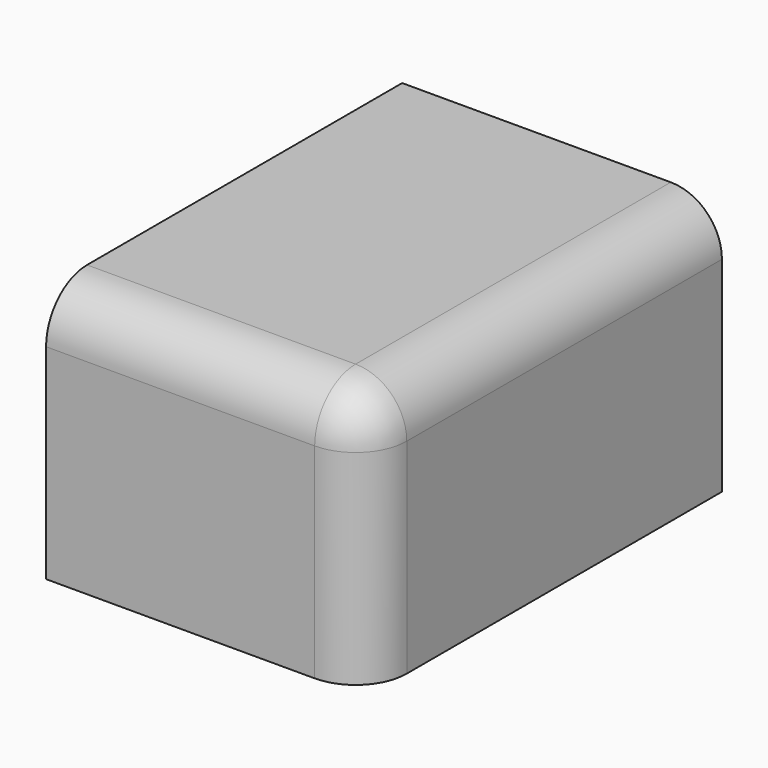
from build123d import *

# Parameters (mm, degrees)
F0_W        = 31.75
F0_H        = 25.4
F1_DEPTH    = 44.196
F2_R        = 5.08
F3_T1_DEPTH = 33.02
F3_S5_W     = 5.08
F3_S5_H     = 5.08
F3_T6_DEPTH = 5.08


# Not quite as in the source:
# - a fillet or chamfer that OpenCascade refuses, or shapes differently, is made with other operations: its cross-section is extruded or revolved along the edge and cut away or added


with BuildPart() as f1:
    # F0 (on Front) → F1 (new body)
    with BuildSketch(Plane.XZ):
        with Locations((3.175, 0)):
            Rectangle(F0_W, F0_H)
    extrude(amount=F1_DEPTH)

    # F2
    f2_edges = [f1.edges().sort_by_distance(p)[0] for p in [
        (3.175, -44.196, 12.7),
        (19.05, -22.098, 12.7),
    ]]
    fillet(f2_edges, radius=F2_R)

    # F3: fillet of radius 5.08 on 1 edges, made by hand

    # F3_s2 → F3_t1 (cut)
    with BuildSketch(Plane.XY.offset(-25.4)):
        with BuildLine():
            ThreePointArc((13.97, -44.196), (17.5621024484, -42.7081024484), (19.05, -39.116))
            Line((19.05, -39.116), (19.05, -44.196))
            Line((19.05, -44.196), (13.97, -44.196))
        make_face()
    extrude(amount=F3_T1_DEPTH, mode=Mode.SUBTRACT)


with BuildPart() as f3_tool4:
    # F3_s5 → F3_t6 (new body)
    with BuildSketch(Plane.XZ.offset(39.116)):
        with Locations((16.51, 10.16)):
            Rectangle(F3_S5_W, F3_S5_H)
    extrude(amount=F3_T6_DEPTH)

    # F3_s7 → F3_t8 (revolve, cut)
    with BuildSketch(Plane(origin=(13.97, -39.116, 7.62), x_dir=(-0.7071067812, 0, -0.7071067812), z_dir=(-0.7071067812, 0, 0.7071067812))):
        with BuildLine():
            ThreePointArc((0, -5.08), (5.08, 0), (0, 5.08))
            Line((0, 5.08), (0, -5.08))
        make_face()
    revolve(axis=Axis((13.97, -39.116, 7.62), (0, -1, 0)), mode=Mode.SUBTRACT)


with BuildPart() as f1_1:
    add(f1.part)

    # F3_t3: cut F3_tool4
    add(f3_tool4.part, mode=Mode.SUBTRACT)


solid = f1_1.part
